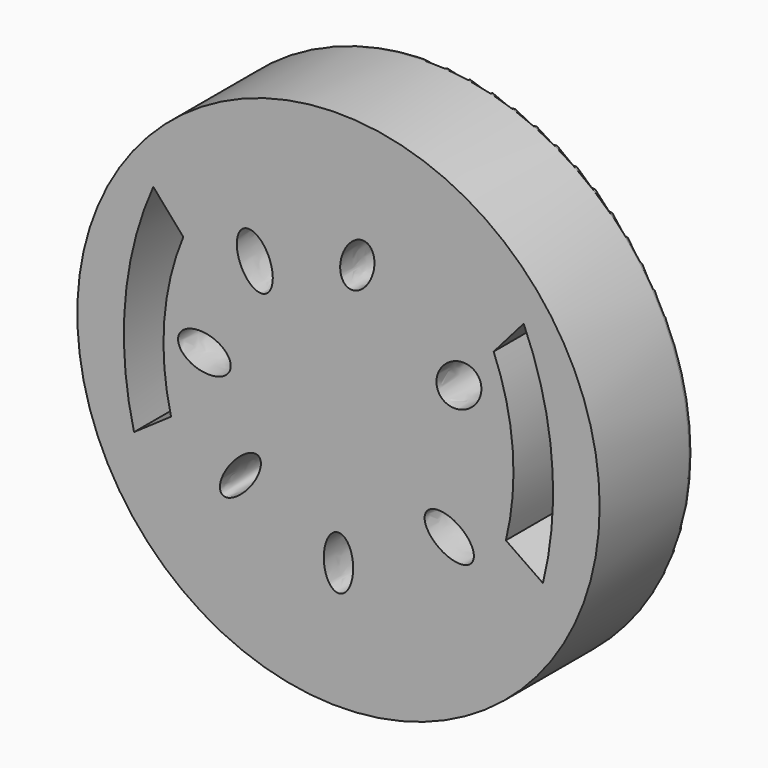
from build123d import *

# Parameters (mm, degrees)
F1_R      = 56.8161487607
F2_DEPTH  = 25.4
F3_R      = 35.5899922612
F3_R_2    = 22.5762653639
F2_FACE_R = 56.8161487607
F4_DEPTH  = 2.54
F6_DEPTH  = 27.94
F7_R      = 7.9040037614
F8_DEPTH  = 4.318
F12_R     = 1.0922


# Not quite as in the source:
# - a fillet or chamfer that OpenCascade refuses, or shapes differently, is made with other operations: its cross-section is extruded or revolved along the edge and cut away or added


with BuildPart() as f2:
    # F1 (on face) → F2 (new body)
    with BuildSketch(Plane.XZ):
        Circle(F1_R)
        with BuildLine():
            ThreePointArc((-44.4710278505, -18.6901881557), (-46.4062188569, 5.8245068962), (-40.2819064718, 29.6406366307))
            Line((-40.2819064718, 29.6406366307), (-33.7583683431, 22.1577528864))
            ThreePointArc((-33.7583683431, 22.1577528864), (-37.9075248121, 4.7276497126), (-36.4142209291, -13.1271546707))
            Line((-36.4142209291, -13.1271546707), (-44.4710278505, -18.6901881557))
        make_face(mode=Mode.SUBTRACT)
        with BuildLine():
            ThreePointArc((36.4142209291, -13.1271546707), (37.9075248121, 4.7276497126), (33.7583683431, 22.1577528864))
            Line((33.7583683431, 22.1577528864), (40.2819064718, 29.6406366307))
            ThreePointArc((40.2819064718, 29.6406366307), (46.4062188569, 5.8245068962), (44.4710278505, -18.6901881557))
            Line((44.4710278505, -18.6901881557), (36.4142209291, -13.1271546707))
        make_face(mode=Mode.SUBTRACT)
    extrude(amount=F2_DEPTH)

    # F3 (on face) + F2_face (on face) → F4 (join)
    with BuildSketch(Plane.XZ):
        Circle(F3_R)
        Circle(F3_R_2, mode=Mode.SUBTRACT)
    with BuildSketch(Plane(origin=(0, -25.4, -0.4063094345), x_dir=(1, 0, 0), z_dir=(0, -1, 0))):
        with Locations((0, 0.4063094345)):
            Circle(F2_FACE_R)
        with BuildLine():
            ThreePointArc((-44.4710278505, -18.2838787212), (-46.4062188569, 6.2308163307), (-40.2819064718, 30.0469460652))
            Line((-40.2819064718, 30.0469460652), (-33.7583683431, 22.5640623209))
            ThreePointArc((-33.7583683431, 22.5640623209), (-37.9075248121, 5.1339591471), (-36.4142209291, -12.7208452362))
            Line((-36.4142209291, -12.7208452362), (-44.4710278505, -18.2838787212))
        make_face(mode=Mode.SUBTRACT)
        with BuildLine():
            Line((33.7583683431, 22.5640623209), (40.2819064718, 30.0469460652))
            ThreePointArc((40.2819064718, 30.0469460652), (46.4062188569, 6.2308163307), (44.4710278505, -18.2838787212))
            Line((44.4710278505, -18.2838787212), (36.4142209291, -12.7208452362))
            ThreePointArc((36.4142209291, -12.7208452362), (37.9075248121, 5.1339591471), (33.7583683431, 22.5640623209))
        make_face(mode=Mode.SUBTRACT)
    extrude(amount=-F4_DEPTH)

    # F5 (on face) → F6 (cut, through all)
    with BuildSketch(Plane(origin=(0, 2.54, 0), x_dir=(-1, 0, 0), z_dir=(0, 1, 0))):
        with BuildLine():
            add(Edge.make_bspline(
                [(-22.1350241453, 9.9253346344), (-17.4387312679, 15.7053885291), (-25.8885159715, 17.7729417092), (-34.3383006751, 19.8404948894), (-30.5848088489, 11.9928878146), (-26.8313170226, 4.1452807398), (-22.1350241453, 9.9253346344)],
                knots=[0, 0, 0, 2.0943951024, 2.0943951024, 4.1887902048, 4.1887902048, 6.2831853072, 6.2831853072, 6.2831853072], degree=2, weights=[1, 0.5, 1, 0.5, 1, 0.5, 1]))
        make_face()
        with BuildLine():
            add(Edge.make_bspline(
                [(-19.1032729127, -13.2813736373), (-22.4317573402, -8.1016355362), (-28.258317075, -15.5050718268), (-34.0848768098, -22.9085081173), (-24.9298326475, -20.6848099278), (-15.7747884853, -18.4611117383), (-19.1032729127, -13.2813736373)],
                knots=[0, 0, 0, 2.0943951024, 2.0943951024, 4.1887902048, 4.1887902048, 6.2831853072, 6.2831853072, 6.2831853072], degree=2, weights=[1, 0.5, 1, 0.5, 1, 0.5, 1]))
        make_face()
        with BuildLine():
            add(Edge.make_bspline(
                [(0, -23.4607158193), (-5.5486157527, -23.4607158193), (-2.7743078764, -32.182005329), (0, -40.9032948387), (2.7743078764, -32.182005329), (5.5486157527, -23.4607158193), (0, -23.4607158193)],
                knots=[0, 0, 0, 2.0943951024, 2.0943951024, 4.1887902048, 4.1887902048, 6.2831853072, 6.2831853072, 6.2831853072], degree=2, weights=[1, 0.5, 1, 0.5, 1, 0.5, 1]))
        make_face()
        with BuildLine():
            add(Edge.make_bspline(
                [(25.2971906755, -24.4050862803), (28.798989351, -21.6016149756), (21.0994370463, -15.5729249819), (13.3998847417, -9.5442349882), (17.5976383709, -18.3763962866), (21.7953920001, -27.208557585), (25.2971906755, -24.4050862803)],
                knots=[0, 0, 0, 2.0943951024, 2.0943951024, 4.1887902048, 4.1887902048, 6.2831853072, 6.2831853072, 6.2831853072], degree=2, weights=[1, 0.5, 1, 0.5, 1, 0.5, 1]))
        make_face()
        with BuildLine():
            add(Edge.make_bspline(
                [(34.8414648329, 2.7295567518), (33.4559524036, 9.1247388108), (25.637388861, 4.0831753651), (17.8188253184, -0.9583880805), (27.0229012903, -2.3120066939), (36.2269772622, -3.6656253073), (34.8414648329, 2.7295567518)],
                knots=[0, 0, 0, 2.0943951024, 2.0943951024, 4.1887902048, 4.1887902048, 6.2831853072, 6.2831853072, 6.2831853072], degree=2, weights=[1, 0.5, 1, 0.5, 1, 0.5, 1]))
        make_face()
        with BuildLine():
            add(Edge.make_bspline(
                [(-6.0858990853, 34.0494873791), (-11.5396176398, 31.868902646), (-5.828270141, 25.4948857644), (-0.1169226421, 19.1208688827), (-0.3745515864, 27.6754704975), (-0.6321805307, 36.2300721122), (-6.0858990853, 34.0494873791)],
                knots=[0, 0, 0, 2.0943951024, 2.0943951024, 4.1887902048, 4.1887902048, 6.2831853072, 6.2831853072, 6.2831853072], degree=2, weights=[1, 0.5, 1, 0.5, 1, 0.5, 1]))
        make_face()
        with BuildLine():
            add(Edge.make_bspline(
                [(20.3246924263, 28.2097336219), (14.6433807466, 30.3649967519), (14.2948588898, 20.8806364475), (13.946337033, 11.396276143), (19.9761705695, 18.7253733174), (26.006004106, 26.0544704918), (20.3246924263, 28.2097336219)],
                knots=[0, 0, 0, 2.0943951024, 2.0943951024, 4.1887902048, 4.1887902048, 6.2831853072, 6.2831853072, 6.2831853072], degree=2, weights=[1, 0.5, 1, 0.5, 1, 0.5, 1]))
        make_face()
    extrude(amount=-F6_DEPTH, mode=Mode.SUBTRACT)

    # F7 (on face) → F8 (join)
    with BuildSketch(Plane.XZ):
        Circle(F7_R)
    extrude(amount=-F8_DEPTH)

    # F9: fillet of radius 5.08 on 1 edges, made by hand

    # F9_s1 → F9_t2 (revolve, cut)
    with BuildSketch(Plane.XY):
        with BuildLine():
            ThreePointArc((7.9040037614, 0), (6.1932337202, 3.0901007256), (2.8814788983, 4.318))
            Line((2.8814788983, 4.318), (2.8814788983, 4.4196))
            Line((2.8814788983, 4.4196), (7.9040037614, 4.4196))
            Line((7.9040037614, 4.4196), (8.0056037614, 4.318))
            ThreePointArc((8.0056037614, 4.318), (8.0056037614, 2.159), (8.0044542586, 0.01524))
            Line((8.0044542586, 0.01524), (7.9040037614, 0))
        make_face()
    revolve(axis=Axis((0, 4.318, 0), (0, -1, 0)), mode=Mode.SUBTRACT)

    # F10: fillet of radius 1.4103835631 on 1 edges, made by hand

    # F10_s1 → F10_t2 (revolve, cut)
    with BuildSketch(Plane.XY):
        with BuildLine():
            ThreePointArc((23.9876146125, 2.5404), (22.9893571455, 2.1269082184), (22.5758653639, 1.1286507514))
            Line((22.5758653639, 1.1286507514), (22.4346904391, 1.1286507514))
            ThreePointArc((22.4346904391, 1.1286507514), (22.4350904391, 1.8343253757), (22.4350904391, 2.54))
            Line((22.4350904391, 2.54), (22.5762653639, 2.6811749249))
            ThreePointArc((22.5762653639, 2.6811749249), (23.2819399882, 2.6811749249), (23.9876146125, 2.6815749249))
            Line((23.9876146125, 2.6815749249), (23.9876146125, 2.5404))
        make_face()
    revolve(axis=Axis((0, 2.54, 0), (0, -1, 0)), mode=Mode.SUBTRACT)

    # F11: fillet of radius 1.1037784407 on 1 edges, made by hand

    # F11_s1 → F11_t2 (revolve, cut)
    with BuildSketch(Plane.XY):
        with BuildLine():
            ThreePointArc((35.5903922612, 1.4352558739), (35.2667030408, 2.2167107796), (34.485248135, 2.5404))
            Line((34.485248135, 2.5404), (34.485248135, 2.6509144126))
            ThreePointArc((34.485248135, 2.6509144126), (35.0376201981, 2.6505144126), (35.5899922612, 2.6505144126))
            Line((35.5899922612, 2.6505144126), (35.7005066738, 2.54))
            ThreePointArc((35.7005066738, 2.54), (35.7005066738, 1.9876279369), (35.7009066738, 1.4352558739))
            Line((35.7009066738, 1.4352558739), (35.5903922612, 1.4352558739))
        make_face()
    revolve(axis=Axis((0, 2.54, 0), (0, -1, 0)), mode=Mode.SUBTRACT)

    # F12
    f12_edges = [f2.edges().sort_by_distance(p)[0] for p in [
        (-56.816149, 0, 0),
    ]]
    fillet(f12_edges, radius=F12_R)


solid = f2.part
